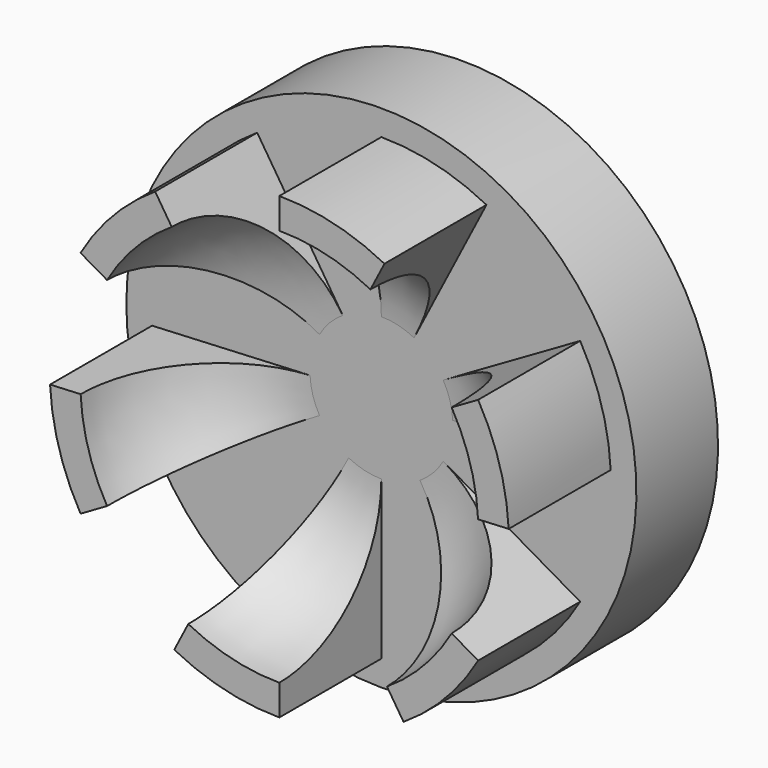
from build123d import *

# Parameters (mm, degrees)
F2_DEPTH        = 5
F2_COPIES_COUNT = 6
F4_R            = 13.5
F5_DEPTH        = 4
F6_R            = 4.99999
F8_DEPTH        = 6
F10_DEPTH       = 1.5
F11_R           = 23.1793955011
F12_DEPTH       = 25


# Not quite as in the source:
# - a fillet or chamfer is up to 0.001 mm smaller than in the source, because OpenCascade refuses the exact size
# - a pattern or mirror of a feature is missing from the dataset's text; its kind, count and spacing are read off the source's solid


with BuildPart() as f2:
    # F1 (on Front) → F2 (new body)
    with BuildSketch(Plane.XZ):
        with BuildLine():
            Line((3.5710217678, 6.9345370094), (4.120409732, 8.001388857))
            ThreePointArc((4.120409732, 8.001388857), (2.1198467265, 8.7467851155), (0, 9))
            Line((0, 9), (0, 7.8))
            ThreePointArc((0, 7.8), (1.8372004963, 7.5805471001), (3.5710217678, 6.9345370094))
        make_face()
    extrude(amount=F2_DEPTH)


with BuildPart() as f2_copies_1:
    # F2_copies: instance of F2
    add(f2.part.rotate(Axis((0, 0, 0), (0, 1, 0)), 1 * 360 / F2_COPIES_COUNT))


with BuildPart() as f2_copies_2:
    # F2_copies: instance of F2
    add(f2.part.rotate(Axis((0, 0, 0), (0, 1, 0)), 2 * 360 / F2_COPIES_COUNT))


with BuildPart() as f2_copies_3:
    # F2_copies: instance of F2
    add(f2.part.rotate(Axis((0, 0, 0), (0, 1, 0)), 3 * 360 / F2_COPIES_COUNT))


with BuildPart() as f2_copies_4:
    # F2_copies: instance of F2
    add(f2.part.rotate(Axis((0, 0, 0), (0, 1, 0)), 4 * 360 / F2_COPIES_COUNT))


with BuildPart() as f2_copies_5:
    # F2_copies: instance of F2
    add(f2.part.rotate(Axis((0, 0, 0), (0, 1, 0)), 5 * 360 / F2_COPIES_COUNT))


with BuildPart() as f2_1:
    add(f2.part)

    add(f2_copies_1.part)  # F5 merges F2_copies_1

    add(f2_copies_2.part)  # F5 merges F2_copies_2

    add(f2_copies_3.part)  # F5 merges F2_copies_3

    add(f2_copies_4.part)  # F5 merges F2_copies_4

    add(f2_copies_5.part)  # F5 merges F2_copies_5
    # F4 (on Front) → F5 (join)
    with BuildSketch(Plane.XZ):
        with Locations((0, 3.5)):
            Circle(F4_R)
    extrude(amount=-F5_DEPTH)

    # F6 (radius 5 in the source; OpenCascade refuses exactly that, so slightly less here)
    f6_edges = [f2_1.edges().sort_by_distance(p)[0] for p in [
        (-1.8372, 0, -7.580547),
        (-7.483547, 0, -2.199211),
        (5.646346, 0, -5.381336),
        (-5.646346, 0, 5.381336),
        (7.483547, 0, 2.199211),
        (1.8372, 0, 7.580547),
    ]]
    fillet(f6_edges, radius=F6_R)

    # F7 (on face) → F8 (join)
    with BuildSketch(Plane.XZ):
        with BuildLine():
            ThreePointArc((-10, 0), (0, 10), (10, 0))
            Line((10, 0), (12, 0))
            ThreePointArc((12, 0), (0, 12), (-12, 0))
            Line((-12, 0), (-10, 0))
        make_face()
    extrude(amount=F8_DEPTH)

    # F9 (on face) → F10 (join)
    with BuildSketch(Plane.XZ.offset(6)):
        with BuildLine():
            Line((12, 0), (13.5, 0))
            ThreePointArc((13.5, 0), (0, 13.5), (-13.5, 0))
            Line((-13.5, 0), (-12, 0))
            ThreePointArc((-12, 0), (0, 12), (12, 0))
        make_face()
        with BuildLine():
            Line((10, 0), (12, 0))
            ThreePointArc((12, 0), (0, 12), (-12, 0))
            Line((-12, 0), (-10, 0))
            ThreePointArc((-10, 0), (0, 10), (10, 0))
        make_face()
    extrude(amount=F10_DEPTH)

    # F11 (on face) → F12 (cut)
    with BuildSketch(Plane(origin=(0, 4, 0), x_dir=(-1, 0, 0), z_dir=(0, 1, 0))):
        Circle(F11_R)
        with BuildLine():
            ThreePointArc((13.5, 3.5), (9.5459415677, -6.0459415243), (6.13e-08, -10))
            ThreePointArc((6.13e-08, -10), (-9.5459415677, 13.0459415243), (13.5, 3.5))
        make_face(mode=Mode.SUBTRACT)
        with BuildLine():
            ThreePointArc((13.5, 3.5), (-9.5459415677, 13.0459415243), (6.13e-08, -10))
            ThreePointArc((6.13e-08, -10), (9.5459415677, -6.0459415243), (13.5, 3.5))
        make_face()
        with BuildLine():
            ThreePointArc((6.13e-08, -10), (-7.0710678335, 7.0710677902), (10, 0))
            ThreePointArc((10, 0), (7.0710678335, -7.0710677902), (6.13e-08, -10))
        make_face(mode=Mode.SUBTRACT)
    extrude(amount=-F12_DEPTH, mode=Mode.SUBTRACT)


solid = f2_1.part
